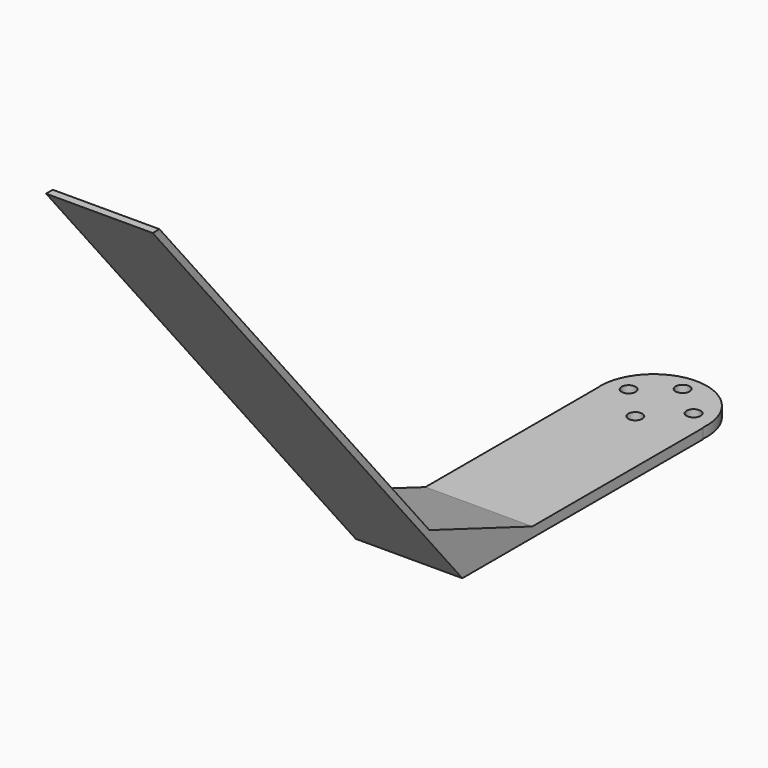
from build123d import *

# Parameters (mm, degrees)
F0_R      = 13.50645
F1_DEPTH  = 2.54
F2_W      = 27.0256
F2_H      = 76.2
F3_DEPTH  = 2.54
F4_R      = 1.778
F5_DEPTH  = 2.541
F7_DEPTH  = 26.9875
F9_DEPTH  = 26.9875
F10_R     = 60.96
F10_W     = 26.9875
F10_H     = 2.1313130632
F11_DEPTH = 50.8
F12_R     = 56.5455680067
F13_DEPTH = 116.7461731313
F15_DEPTH = 50.801
F17_DEPTH = 50.8
F19_DEPTH = 25.4
F20_DEPTH = 26.9875
F21_DEPTH = 25.4


# Not quite as in the source:
# - a feature names something its author has since deleted; it is built from what else it names


with BuildPart() as f1:
    # F0 (on Top) → F1 (new body)
    with BuildSketch(Plane.XY):
        with Locations((0, 38.9145108197)):
            Circle(F0_R)
    extrude(amount=F1_DEPTH)

    # F2 (on Top) → F3 (join)
    with BuildSketch(Plane.XY):
        with Locations((0.0679422232, -0.4738955459)):
            Rectangle(F2_W, F2_H)
    extrude(amount=F3_DEPTH)

    # F4 (on Top) → F5 (cut, through all)
    with BuildSketch(Plane.XY):
        with Locations((-8.2149387259, 41.2970071224)):
            Circle(F4_R)
        with Locations((0, 48.1029608197)):
            Circle(F4_R)
        with Locations((0, 33.1169608197)):
            Circle(F4_R)
        with Locations((8.2149387259, 41.2970071224)):
            Circle(F4_R)
    extrude(amount=F5_DEPTH, mode=Mode.SUBTRACT)

    # F6 (on face) → F7 (join)
    with BuildSketch(Plane.YZ.offset(13.5807422232)):
        Polygon((-136.5347272621, 116.7451731313), (-38.5738955459, 0), (-38.5738955459, 2.54), (-134.4034141989, 116.7451731313), align=None)
    extrude(amount=-F7_DEPTH)

    # F8 (on face) → F9 (join)
    with BuildSketch(Plane(origin=(-13.4067577768, 0, 0), x_dir=(0, -1, 0), z_dir=(-1, 0, 0))):
        Polygon((38.5738955459, 2.54), (49.0018958172, 14.9676067869), (16.4343814087, 2.54), align=None)
    extrude(amount=-F9_DEPTH)


with BuildPart() as f11:
    # F10 (on face) → F11 (new body)
    with BuildSketch(Plane.XY.offset(116.7451731313)):
        with Locations((0, -175.3809303045)):
            Circle(F10_R)
        with Locations((0.0869922232, -135.4690707305)):
            Rectangle(F10_W, F10_H, mode=Mode.SUBTRACT)
    extrude(amount=-F11_DEPTH)

    # F12 (on face) → F13 (cut, through all)
    with BuildSketch(Plane.XY.offset(116.7451731313)):
        with Locations((-8.7670916691, -175.4986345768)):
            Circle(F12_R)
    extrude(amount=-F13_DEPTH, mode=Mode.SUBTRACT)

    # F14 (on face) → F15 (cut, through all)
    with BuildSketch(Plane(origin=(0, 0, 65.9451731313), x_dir=(1, 0, 0), z_dir=(0, 0, -1))):
        with BuildLine():
            ThreePointArc((-34.6411562373, 125.2200701191), (-26.8424040995, 120.6487921939), (-18.4533903647, 117.2810681356))
            Line((-18.4533903647, 117.2810681356), (-18.4533903647, 119.7888788891))
            ThreePointArc((-18.4533903647, 119.7888788891), (-26.7534564605, 121.8899417854), (-34.6411562373, 125.2200701191))
        make_face()
    extrude(amount=-F15_DEPTH, mode=Mode.SUBTRACT)

    # F16 (on face) → F17 (cut)
    with BuildSketch(Plane(origin=(0, 0, 65.9451731313), x_dir=(1, 0, 0), z_dir=(0, 0, -1))):
        with BuildLine():
            Line((-12.9449410231, 231.889651911), (-12.9449410231, 234.9506382265))
            ThreePointArc((-12.9449410231, 234.9506382265), (-23.5006925786, 231.6289440324), (-33.2820246218, 226.4537061942))
            ThreePointArc((-33.2820246218, 226.4537061942), (-23.3686777331, 230.1264200492), (-12.9449410231, 231.889651911))
        make_face()
    extrude(amount=-F17_DEPTH, mode=Mode.SUBTRACT)


with BuildPart() as f19:
    # F18 (on face) → F19 (new body)
    with BuildSketch(Plane(origin=(-13.4067577768, 0, 0), x_dir=(0, -1, 0), z_dir=(-1, 0, 0))):
        Polygon((116.024311172, 92.3018110703), (105.3223571677, 79.5477189379), (117.2810681356, 79.5477189379), align=None)
    extrude(amount=F19_DEPTH)


with BuildPart() as f20:
    # F18 (on face) → F20 (new body)
    with BuildSketch(Plane(origin=(-13.4067577768, 0, 0), x_dir=(0, -1, 0), z_dir=(-1, 0, 0))):
        Polygon((116.024311172, 92.3018110703), (105.3223571677, 79.5477189379), (117.2810681356, 79.5477189379), align=None)
    extrude(amount=-F20_DEPTH)


with BuildPart() as f21_tool:
    # F21 (cut): a face of the model
    f21_faces = [f19.part.faces().sort_by_distance(p)[0] for p in [
        (-38.8067577768, -112.8759121584, 83.7990829821),
    ]]
    extrude(f21_faces, amount=-F21_DEPTH)


with BuildPart() as f11_1:
    add(f11.part)

    # F21: cut by f21_tool
    add(f21_tool.part, mode=Mode.SUBTRACT)


with BuildPart() as f19_1:
    add(f19.part)

    # F21: cut by f21_tool
    add(f21_tool.part, mode=Mode.SUBTRACT)


solid = f1.part
